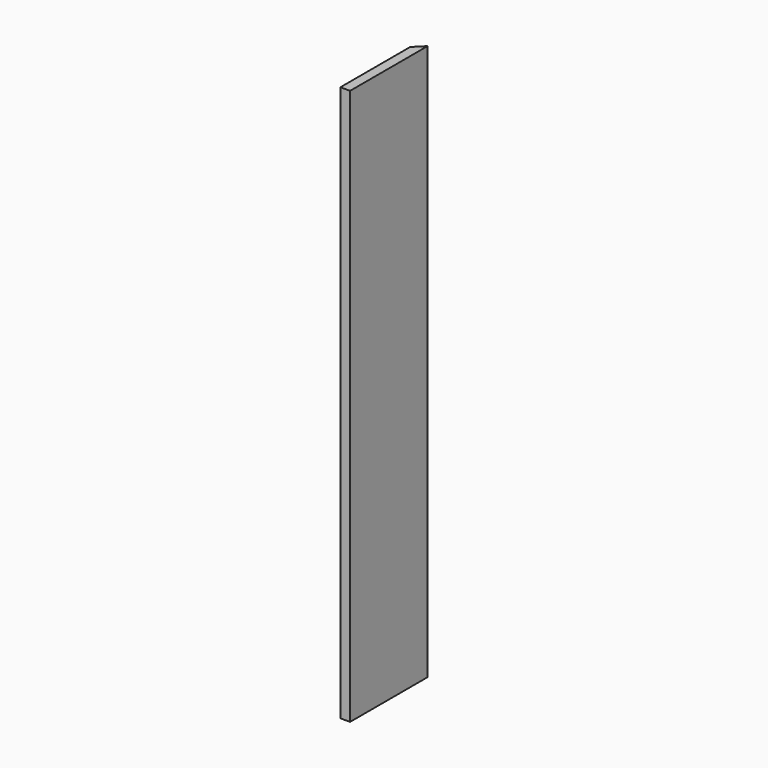
from build123d import *

# Parameters (mm, degrees)
F0_W     = 190.5
F0_H     = 1092.2
F1_DEPTH = 19.05
F2_SIZE  = 19.04999


# Not quite as in the source:
# - a fillet or chamfer is up to 0.001 mm smaller than in the source, because OpenCascade refuses the exact size


with BuildPart() as f1:
    # F0 (on Right) → F1 (new body)
    with BuildSketch(Plane.YZ):
        Rectangle(F0_W, F0_H)
    extrude(amount=F1_DEPTH)

    # F2 (size 19.05 in the source; OpenCascade refuses exactly that, so slightly less here)
    f2_edges = [f1.edges().sort_by_distance(p)[0] for p in [
        (0, 95.25, 0),
    ]]
    chamfer(f2_edges, length=F2_SIZE)


solid = f1.part
